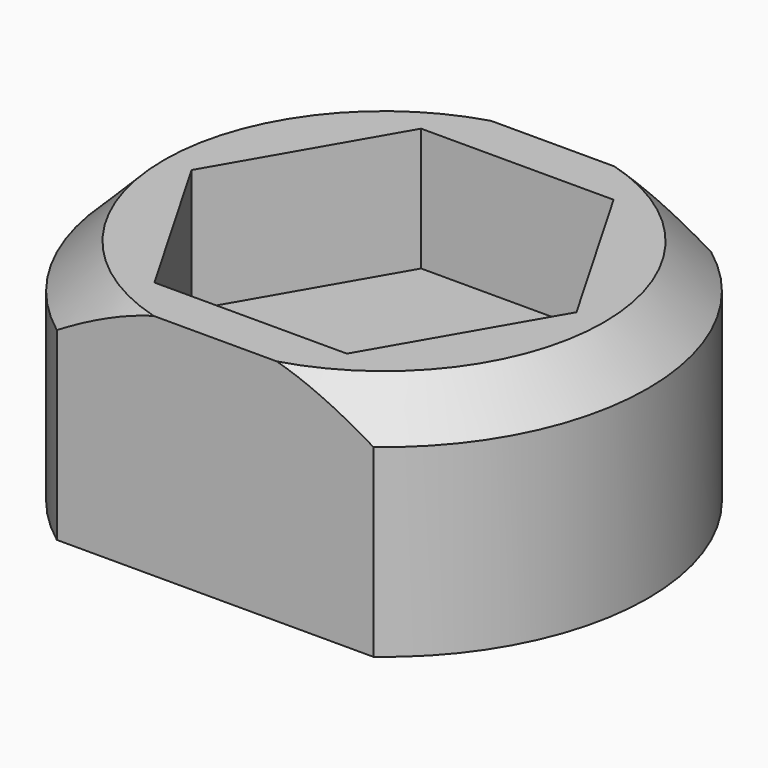
from build123d import *

# Parameters (mm, degrees)
F1_DEPTH = 13
F3_DEPTH = 7
F4_SIZE  = 2.5
F5_DEPTH = 2


# Not quite as in the source:
# - a feature names something its author has since deleted; it is built from what else it names


with BuildPart() as f1:
    # F0 (on Top) → F1 (new body)
    with BuildSketch(Plane.XY):
        with BuildLine():
            ThreePointArc((9, -12), (13.416407865, -6.7082039325), (15, 0))
            ThreePointArc((15, 0), (13.416407865, 6.7082039325), (9, 12))
            Line((9, 12), (-9, 12))
            ThreePointArc((-9, 12), (-15, 0), (-9, -12))
            Line((-9, -12), (9, -12))
        make_face()
    extrude(amount=F1_DEPTH)

    # F2 (on face) → F3 (cut)
    with BuildSketch(Plane.XY.offset(13)):
        Polygon((5.4703938006, -9.475), (10.9407876011, 0), (5.4703938006, 9.475), (-5.4703938006, 9.475), (-10.9407876011, 0), (-5.4703938006, -9.475), align=None)
    extrude(amount=-F3_DEPTH, mode=Mode.SUBTRACT)

    # F4
    f4_edges = [f1.edges().sort_by_distance(p)[0] for p in [
        (15, 0, 13),
        (-15, 0, 13),
    ]]
    chamfer(f4_edges, length=F4_SIZE)

    # F0 (on Top) → F5 (join)
    with BuildSketch(Plane.XY):
        with BuildLine():
            ThreePointArc((9, -12), (13.416407865, -6.7082039325), (15, 0))
            ThreePointArc((15, 0), (13.416407865, 6.7082039325), (9, 12))
            Line((9, 12), (-9, 12))
            ThreePointArc((-9, 12), (-15, 0), (-9, -12))
            Line((-9, -12), (9, -12))
        make_face()
    extrude(amount=F5_DEPTH)


solid = f1.part
